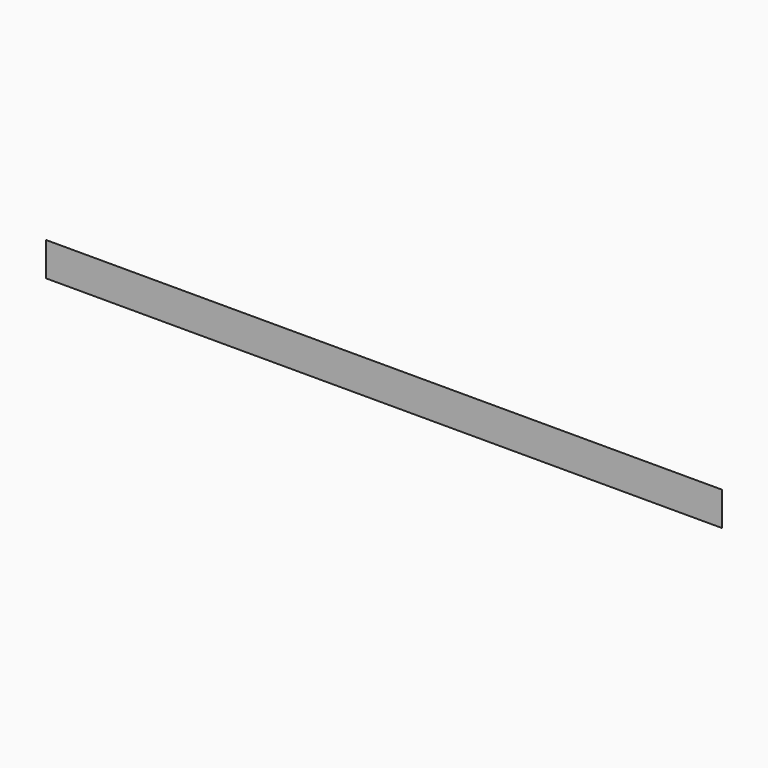
from build123d import *

# Parameters (mm, degrees)
F0_W     = 1500
F0_H     = 75
F1_DEPTH = 12
F2_SIZE  = 11.99999


# Not quite as in the source:
# - a fillet or chamfer is up to 0.001 mm smaller than in the source, because OpenCascade refuses the exact size


with BuildPart() as f1:
    # F0 (on Front) → F1 (new body)
    with BuildSketch(Plane.XZ):
        Rectangle(F0_W, F0_H)
    extrude(amount=F1_DEPTH)

    # F2 (size 12 in the source; OpenCascade refuses exactly that, so slightly less here)
    f2_edges = [f1.edges().sort_by_distance(p)[0] for p in [
        (0, 0, 37.5),
        (750, 0, 0),
        (-750, 0, 0),
    ]]
    chamfer(f2_edges, length=F2_SIZE)


solid = f1.part
